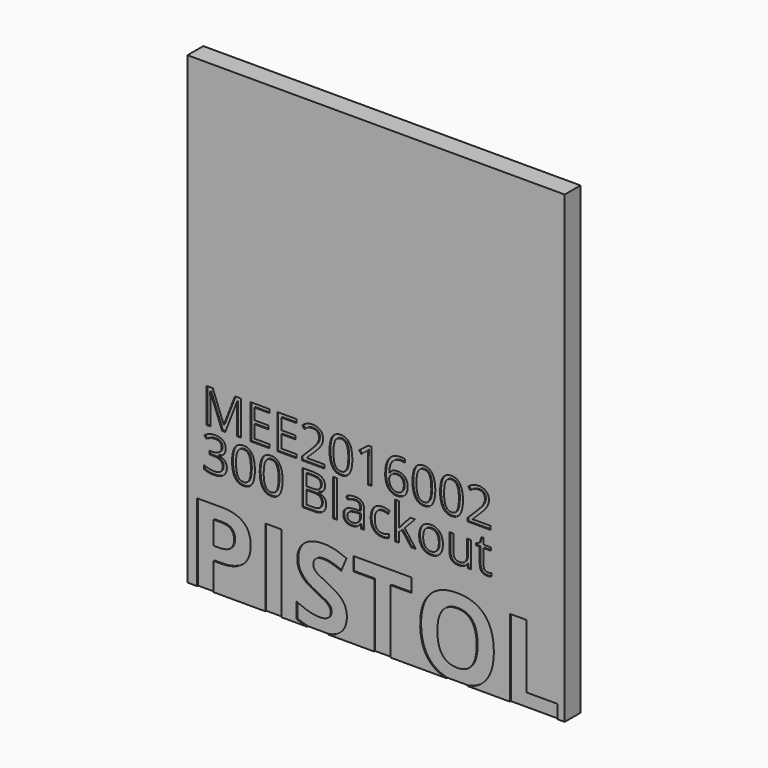
from build123d import *

# Parameters (mm, degrees)
F0_W         = 41.275
F0_H         = 50.8
F1_DEPTH     = 2.159
F2_TEXT_SIZE = 11.8590347924
F3_DEPTH     = 0.127
F4_TEXT_SIZE = 5.2916666667
F5_DEPTH     = 0.127
F6_TEXT_SIZE = 5.2916666667
F7_DEPTH     = 0.127


# Not quite as in the source:
# - Text() gives the source's letters only with a copy of the font that has no kerning and outlines rounded to 1/6400 em; it was checked with that copy


with BuildPart() as f1:
    # F0 (on Front) → F1 (new body)
    with BuildSketch(Plane.XZ):
        with Locations((20.6375, 25.4)):
            Rectangle(F0_W, F0_H)
    extrude(amount=-F1_DEPTH)

    # F2 (on face) → F3 (cut)
    with BuildSketch(Plane.XZ):
        with Locations((0, 0)):
            Text('PISTOL', F2_TEXT_SIZE, font='Open Sans', font_style=FontStyle.BOLD, text_align=(TextAlign.LEFT, TextAlign.BOTTOM))
    extrude(amount=-F3_DEPTH, mode=Mode.SUBTRACT)

    # F4 (on Front) → F5 (cut)
    with BuildSketch(Plane.XZ):
        with Locations((1.5875, 15.8508986671)):
            Text('MEE2016002', F4_TEXT_SIZE, font='Open Sans', text_align=(TextAlign.LEFT, TextAlign.BOTTOM))
    extrude(amount=-F5_DEPTH, mode=Mode.SUBTRACT)

    # F6 (on face) → F7 (cut)
    with BuildSketch(Plane.XZ):
        with Locations((1.5875, 11.3579958852)):
            Text('300 Blackout', F6_TEXT_SIZE, font='Open Sans', text_align=(TextAlign.LEFT, TextAlign.BOTTOM))
    extrude(amount=-F7_DEPTH, mode=Mode.SUBTRACT)


solid = f1.part
